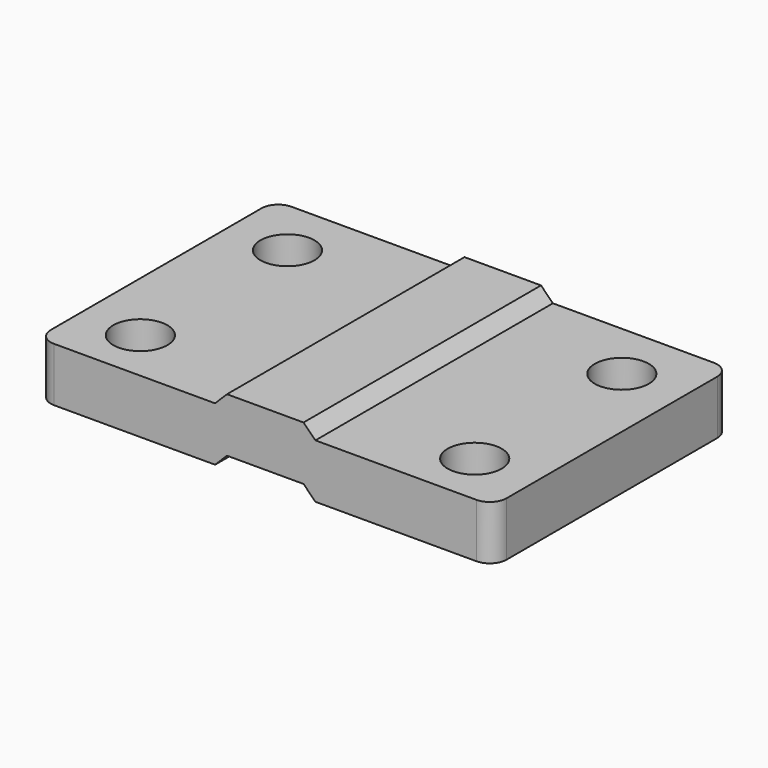
from build123d import *

# Parameters (mm, degrees)
F0_W     = 136.31
F0_H     = 16.17
F1_DEPTH = 88.79
F3_DEPTH = 88.79
F5_DEPTH = 88.79
F6_R     = 5
F8_D     = 16.17


with BuildPart() as f1:
    # F0 (on Front) → F1 (new body)
    with BuildSketch(Plane.XZ):
        with Locations((0, 8.085)):
            Rectangle(F0_W, F0_H)
    extrude(amount=-F1_DEPTH)

    # F2 (on face) → F3 (join)
    with BuildSketch(Plane.XZ):
        Polygon((-15, 16.17), (0, 16.17), (15, 16.17), (11.445, 19.725), (-11.445, 19.725), align=None)
    extrude(amount=-F3_DEPTH)

    # F4 (on Front) → F5 (cut)
    with BuildSketch(Plane.XZ):
        Polygon((-15, 0), (0, 0), (15, 0), (11.4644660941, 3.5355339059), (-11.4644660941, 3.5355339059), align=None)
    extrude(amount=-F5_DEPTH, mode=Mode.SUBTRACT)

    # F6
    f6_edges = [f1.edges().sort_by_distance(p)[0] for p in [
        (68.155, 88.79, 8.085),
        (-68.155, 88.79, 8.085),
        (68.155, 0, 8.085),
        (-68.155, 0, 8.085),
    ]]
    fillet(f6_edges, radius=F6_R)

    # F8 (through all)
    with Locations(Plane(origin=(0, 0, 0), x_dir=(1, 0, 0), z_dir=(0, 0, -1))):
        with Locations((-50.155, -71), (-50.155, -16), (49.845, -71), (49.845, -16)):
            Hole(F8_D / 2)


solid = f1.part
